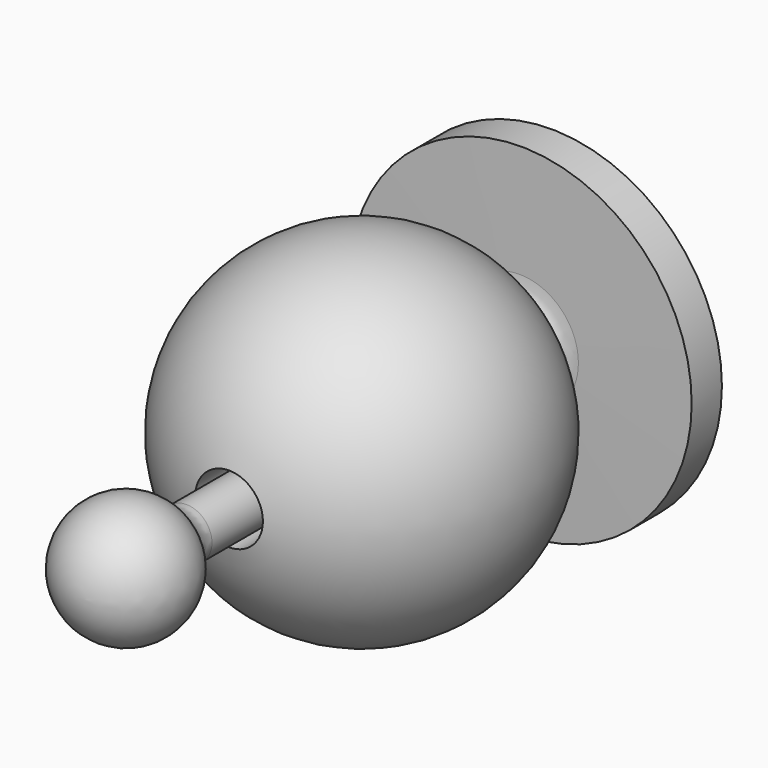
from build123d import *

# Parameters (mm, degrees)
F3_R = 5


with BuildPart() as f1:
    # F0 (on Top) → F1 (revolve)
    with BuildSketch(Plane.XY):
        with BuildLine():
            Line((5, 24.4948974278), (5, -24.4948974278))
            ThreePointArc((5, -24.4948974278), (25, 0), (5, 24.4948974278))
        make_face()
    revolve(axis=Axis((0, 0, 0), (0, -1, 0)))


with BuildPart() as f2:
    # F0 (on Top) → F2 (revolve)
    with BuildSketch(Plane.XY):
        with BuildLine():
            Line((0, 34.9416658282), (0, 25))
            Line((0, 25), (0, -25))
            Line((0, -25), (0, -43.5546562076))
            Line((0, -43.5546562076), (0, -52.7815136387))
            ThreePointArc((0, -52.7815136387), (9.0236258557, -45.4805519658), (3.7669516169, -35.1317722851))
            Line((3.7669516169, -35.1317722851), (3.7669516169, 29.0384795517))
            Line((3.7669516169, 29.0384795517), (25.2225138247, 29.3609593064))
            Line((25.2225138247, 29.3609593064), (25.2225138247, 34.9416658282))
            Line((25.2225138247, 34.9416658282), (0, 34.9416658282))
        make_face()
    revolve(axis=Axis((0, 0, 0), (0, -1, 0)))

    # F3
    f3_edges = [f2.edges().sort_by_distance(p)[0] for p in [
        (-3.766952, 29.03848, 0),
        (-3.766952, -35.131772, 0),
    ]]
    fillet(f3_edges, radius=F3_R)


solid = Compound([f1.part, f2.part])
